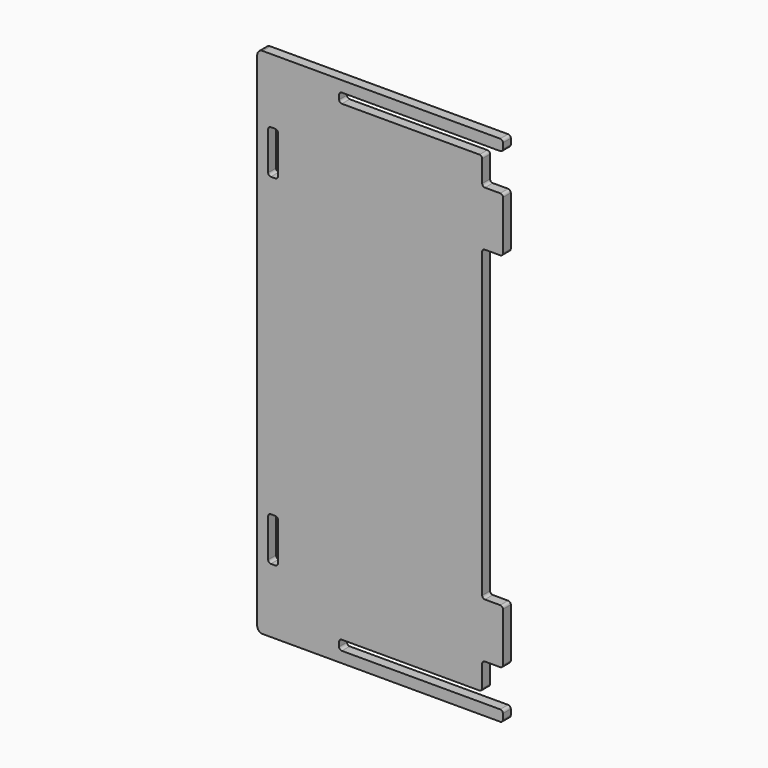
from build123d import *

# Parameters (mm, degrees)
F1_DEPTH = 18
F2_W     = 18
F2_H     = 80
F3_DEPTH = 25
F4_R     = 10
F5_R     = 5
F6_R     = 5
F7_R     = 5


# Not quite as in the source:
# - two fillets or chamfers of one size are made in one step


with BuildPart() as f1:
    # F0 (on Front) → F1 (new body)
    with BuildSketch(Plane.XZ):
        Polygon((0, 940), (0, 0), (450, 0), (450, 20), (150, 20), (150, 38), (412, 38), (412, 88), (450, 88), (450, 188), (412, 188), (412, 752), (450, 752), (450, 852), (412, 852), (412, 902), (150, 902), (150, 920), (450, 920), (450, 940), align=None)
    extrude(amount=F1_DEPTH)

    # F2 (on face) → F3 (cut)
    with BuildSketch(Plane.XZ.offset(18)):
        with Locations((29, 782)):
            Rectangle(F2_W, F2_H)
        with Locations((29, 158)):
            Rectangle(F2_W, F2_H)
    extrude(amount=-F3_DEPTH, mode=Mode.SUBTRACT)

    # F4
    f4_edges = [f1.edges().sort_by_distance(p)[0] for p in [
        (0, -9, 0),
        (0, -9, 940),
    ]]
    fillet(f4_edges, radius=F4_R)

    # F5
    f5_edges = [f1.edges().sort_by_distance(p)[0] for p in [
        (20, -9, 822),
        (38, -9, 822),
        (20, -9, 742),
        (38, -9, 742),
    ]]
    fillet(f5_edges, radius=F5_R)

    # F6
    f6_edges = [f1.edges().sort_by_distance(p)[0] for p in [
        (38, -9, 198),
        (20, -9, 198),
        (20, -9, 118),
        (38, -9, 118),
    ]]
    fillet(f6_edges, radius=F6_R)

    # F7
    f7_edges = [f1.edges().sort_by_distance(p)[0] for p in [
        (450, -9, 0),
        (450, -9, 20),
        (150, -9, 38),
        (150, -9, 20),
        (450, -9, 940),
        (450, -9, 920),
        (150, -9, 920),
        (150, -9, 902),
        (412, -9, 902),
        (412, -9, 38),
        (412, -9, 852),
        (412, -9, 88),
        (450, -9, 852),
        (450, -9, 88),
        (450, -9, 752),
        (450, -9, 188),
        (412, -9, 752),
        (412, -9, 188),
    ]]
    fillet(f7_edges, radius=F7_R)


solid = f1.part
